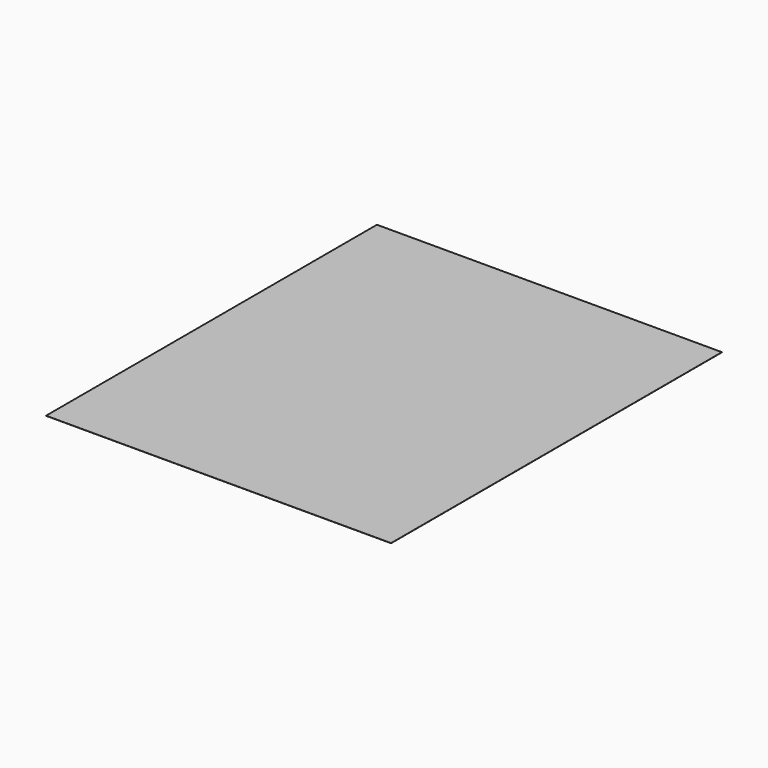
from build123d import *

# Parameters (mm, degrees)
F0_W     = 3708.4
F0_H     = 4445
F1_DEPTH = 1.5875


# Not quite as in the source:
# - a length typed as a fraction of an inch, garbled in the dataset ("3 / 203.2 mm" for 3/8 in), is restored


with BuildPart() as f1:
    # F0 (on Top) → F1 (new body)
    with BuildSketch(Plane.XY):
        with Locations((1854.2, 2222.5)):
            Rectangle(F0_W, F0_H)
    extrude(amount=F1_DEPTH)


solid = f1.part
